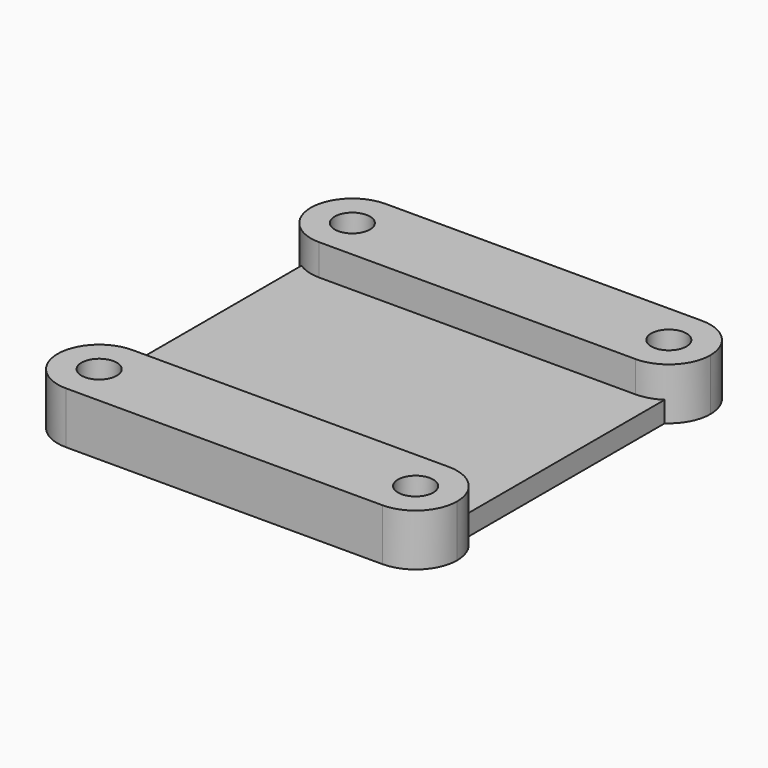
from build123d import *

# Parameters (mm, degrees)
F0_W     = 35
F0_H     = 22.5
F1_DEPTH = 2
F0_R     = 1.7
F2_DEPTH = 5
F3_R     = 4
F3_R_2   = 3.99999
F4_R     = 3
F5_DEPTH = 3


# Not quite as in the source:
# - a fillet or chamfer is up to 0.001 mm smaller than in the source, because OpenCascade refuses the exact size


with BuildPart() as f1:
    # F0 (on Top) → F1 (new body)
    with BuildSketch(Plane.XY):
        Rectangle(F0_W, F0_H)
    extrude(amount=F1_DEPTH)

    # F0 (on Top) → F2 (join)
    with BuildSketch(Plane.XY):
        Polygon((-19.25, -11.25), (-19.25, -19.25), (19.25, -19.25), (19.25, -11.25), (17.5, -11.25), (-17.5, -11.25), align=None)
        with Locations((-15.25, -15.25)):
            Circle(F0_R, mode=Mode.SUBTRACT)
        with Locations((15.25, -15.25)):
            Circle(F0_R, mode=Mode.SUBTRACT)
        Polygon((-19.25, 19.25), (-19.25, 11.25), (-17.5, 11.25), (17.5, 11.25), (19.25, 11.25), (19.25, 19.25), align=None)
        with Locations((-15.25, 15.25)):
            Circle(F0_R, mode=Mode.SUBTRACT)
        with Locations((15.25, 15.25)):
            Circle(F0_R, mode=Mode.SUBTRACT)
    extrude(amount=F2_DEPTH)

    # F3 (call 1 of 8: OpenCascade refuses the feature's edges together)
    f3_edges = [f1.edges().sort_by_distance(p)[0] for p in [
        (19.25, -19.25, 2.5),
    ]]
    fillet(f3_edges, radius=F3_R)

    # F3#2 (call 2 of 8) (radius 4 in the source; OpenCascade refuses exactly that, so slightly less here)
    f3_2_edges = [f1.edges().sort_by_distance(p)[0] for p in [
        (19.25, -11.25, 2.5),
    ]]
    fillet(f3_2_edges, radius=F3_R_2)

    # F3#3 (call 3 of 8)
    f3_3_edges = [f1.edges().sort_by_distance(p)[0] for p in [
        (-19.25, -19.25, 2.5),
    ]]
    fillet(f3_3_edges, radius=F3_R)

    # F3#4 (call 4 of 8)
    f3_4_edges = [f1.edges().sort_by_distance(p)[0] for p in [
        (-19.25, 11.25, 2.5),
    ]]
    fillet(f3_4_edges, radius=F3_R)

    # F3#5 (call 5 of 8)
    f3_5_edges = [f1.edges().sort_by_distance(p)[0] for p in [
        (19.25, 11.25, 2.5),
    ]]
    fillet(f3_5_edges, radius=F3_R)

    # F3#6 (call 6 of 8) (radius 4 in the source; OpenCascade refuses exactly that, so slightly less here)
    f3_6_edges = [f1.edges().sort_by_distance(p)[0] for p in [
        (19.25, 19.25, 2.5),
    ]]
    fillet(f3_6_edges, radius=F3_R_2)

    # F3#7 (call 7 of 8) (radius 4 in the source; OpenCascade refuses exactly that, so slightly less here)
    f3_7_edges = [f1.edges().sort_by_distance(p)[0] for p in [
        (-19.25, -11.25, 2.5),
    ]]
    fillet(f3_7_edges, radius=F3_R_2)

    # F3#8 (call 8 of 8) (radius 4 in the source; OpenCascade refuses exactly that, so slightly less here)
    f3_8_edges = [f1.edges().sort_by_distance(p)[0] for p in [
        (-19.25, 19.25, 2.5),
    ]]
    fillet(f3_8_edges, radius=F3_R_2)

    # F4 (on face) → F5 (cut)
    with BuildSketch(Plane.XY):
        with Locations((-15.25, -15.25)):
            Circle(F4_R)
        with Locations((15.25, -15.25)):
            Circle(F4_R)
        with Locations((15.25, 15.25)):
            Circle(F4_R)
        with Locations((-15.25, 15.25)):
            Circle(F4_R)
    extrude(amount=F5_DEPTH, mode=Mode.SUBTRACT)


solid = f1.part
